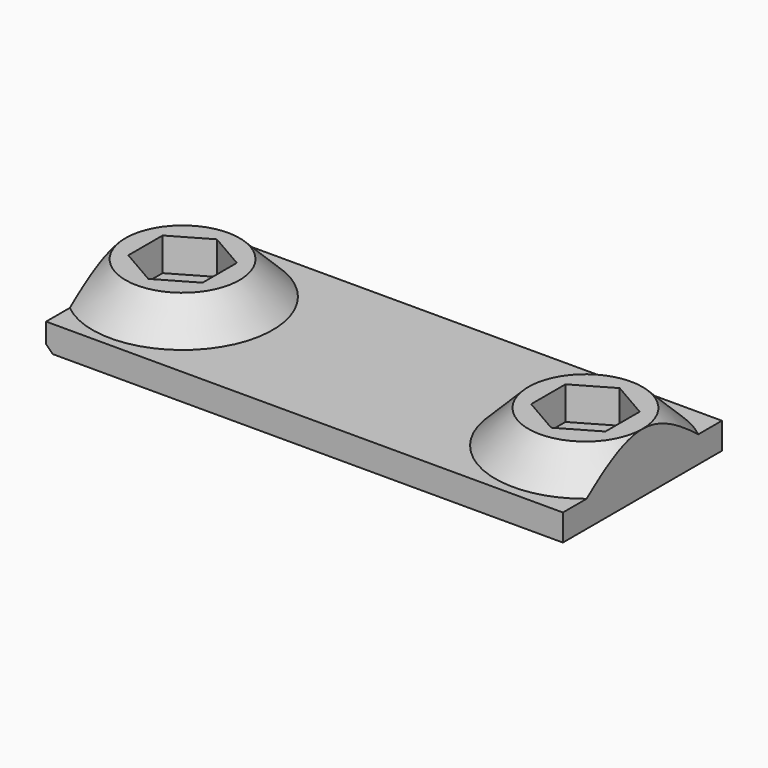
from build123d import *

# Parameters (mm, degrees)
F0_R     = 4.3
F1_DEPTH = 2
F2_D     = 2.85
F2_DEPTH = 11
F2_TIP   = 0.8562263821
F3_DEPTH = 2.5
F5_SIZE  = 0.5


# Not quite as in the source:
# - a fillet or chamfer that OpenCascade refuses, or shapes differently, is made with other operations: its cross-section is extruded or revolved along the edge and cut away or added


with BuildPart() as f1:
    # F0 (on Top) → F1 (new body)
    with BuildSketch(Plane.XY):
        Polygon((-24.6178394498, -8.8684120262), (-63.6178394498, -8.8684120262), (-63.6178394498, -16.3684120262), (-63.6178394498, -23.8684120262), (-24.6178394498, -23.8684120262), (-24.6178394498, -16.3684120262), align=None)
        with BuildLine():
            ThreePointArc((-55.0178394498, -16.3684120262), (-59.3178394498, -20.6684120262), (-63.6178394498, -16.3684120262))
            ThreePointArc((-63.6178394498, -16.3684120262), (-59.3178394498, -12.0684120262), (-55.0178394498, -16.3684120262))
        make_face(mode=Mode.SUBTRACT)
        with Locations((-28.9178394498, -16.3684120262)):
            Circle(F0_R, mode=Mode.SUBTRACT)
        with BuildLine():
            ThreePointArc((-55.0178394498, -16.3684120262), (-59.3178394498, -12.0684120262), (-63.6178394498, -16.3684120262))
            ThreePointArc((-63.6178394498, -16.3684120262), (-59.3178394498, -20.6684120262), (-55.0178394498, -16.3684120262))
        make_face()
        Polygon((-59.3178394498, -13.1352505188), (-56.5178394498, -14.7518312725), (-56.5178394498, -17.98499278), (-59.3178394498, -19.6015735337), (-62.1178394498, -17.98499278), (-62.1178394498, -14.7518312725), align=None, mode=Mode.SUBTRACT)
        with Locations((-28.9178394498, -16.3684120262)):
            Circle(F0_R)
        Polygon((-28.9178394498, -13.1352505188), (-26.1178394498, -14.7518312725), (-26.1178394498, -17.98499278), (-28.9178394498, -19.6015735337), (-31.7178394498, -17.98499278), (-31.7178394498, -14.7518312725), align=None, mode=Mode.SUBTRACT)
        Polygon((-56.5178394498, -17.98499278), (-56.5178394498, -14.7518312725), (-59.3178394498, -13.1352505188), (-62.1178394498, -14.7518312725), (-62.1178394498, -17.98499278), (-59.3178394498, -19.6015735337), align=None)
        Polygon((-26.1178394498, -17.98499278), (-26.1178394498, -14.7518312725), (-28.9178394498, -13.1352505188), (-31.7178394498, -14.7518312725), (-31.7178394498, -17.98499278), (-28.9178394498, -19.6015735337), align=None)
    extrude(amount=-F1_DEPTH)

    # F2
    with Locations(Plane.XY):
        with Locations((-59.3178394498, -16.3684120262), (-28.9178394498, -16.3684120262)):
            Hole(F2_D / 2, depth=F2_DEPTH)
            with Locations((0, 0, -(F2_DEPTH + F2_TIP / 2))):  # 118° drill point
                Cone(0, F2_D / 2, F2_TIP, mode=Mode.SUBTRACT)

    # F0 (on Top) → F3 (join)
    with BuildSketch(Plane.XY):
        with BuildLine():
            ThreePointArc((-55.0178394498, -16.3684120262), (-59.3178394498, -12.0684120262), (-63.6178394498, -16.3684120262))
            ThreePointArc((-63.6178394498, -16.3684120262), (-59.3178394498, -20.6684120262), (-55.0178394498, -16.3684120262))
        make_face()
        Polygon((-59.3178394498, -13.1352505188), (-56.5178394498, -14.7518312725), (-56.5178394498, -17.98499278), (-59.3178394498, -19.6015735337), (-62.1178394498, -17.98499278), (-62.1178394498, -14.7518312725), align=None, mode=Mode.SUBTRACT)
        with Locations((-28.9178394498, -16.3684120262)):
            Circle(F0_R)
        Polygon((-28.9178394498, -13.1352505188), (-26.1178394498, -14.7518312725), (-26.1178394498, -17.98499278), (-28.9178394498, -19.6015735337), (-31.7178394498, -17.98499278), (-31.7178394498, -14.7518312725), align=None, mode=Mode.SUBTRACT)
    extrude(amount=F3_DEPTH)

    # F4: chamfer of 2.5 on 2 edges, made by hand


with BuildPart() as f4_tool2:
    # F4_s3 → F4_t4 (revolve)
    with BuildSketch(Plane.XZ.offset(16.3684120262)):
        Polygon((-66.1178394498, 0), (-63.6178394498, 2.5), (-63.6178394498, 0), align=None)
    revolve(axis=Axis((-59.3178394498, -16.3684120262, 0), (0, 0, 1)))

    split(bisect_by=Plane.YZ.offset(-63.6178394498), keep=Keep.TOP)


with BuildPart() as f1_1:
    add(f1.part)

    # F4_t1: union F4_tool2
    add(f4_tool2.part)


with BuildPart() as f4_tool7:
    # F4_s8 → F4_t9 (revolve)
    with BuildSketch(Plane.XZ.offset(16.3684120262)):
        Polygon((-22.1178394498, 0), (-24.6178394498, 2.5), (-24.6178394498, 0), align=None)
    revolve(axis=Axis((-28.9178394498, -16.3684120262, 0), (0, 0, 1)))

    split(bisect_by=Plane.YZ.offset(-24.6178394498), keep=Keep.BOTTOM)


with BuildPart() as f1_2:
    add(f1_1.part)

    # F4_t6: union F4_tool7
    add(f4_tool7.part)

    # F5
    f5_edges = [f1_2.edges().sort_by_distance(p)[0] for p in [
        (-63.617839, -16.368412, -2),
    ]]
    chamfer(f5_edges, length=F5_SIZE)


solid = f1_2.part
